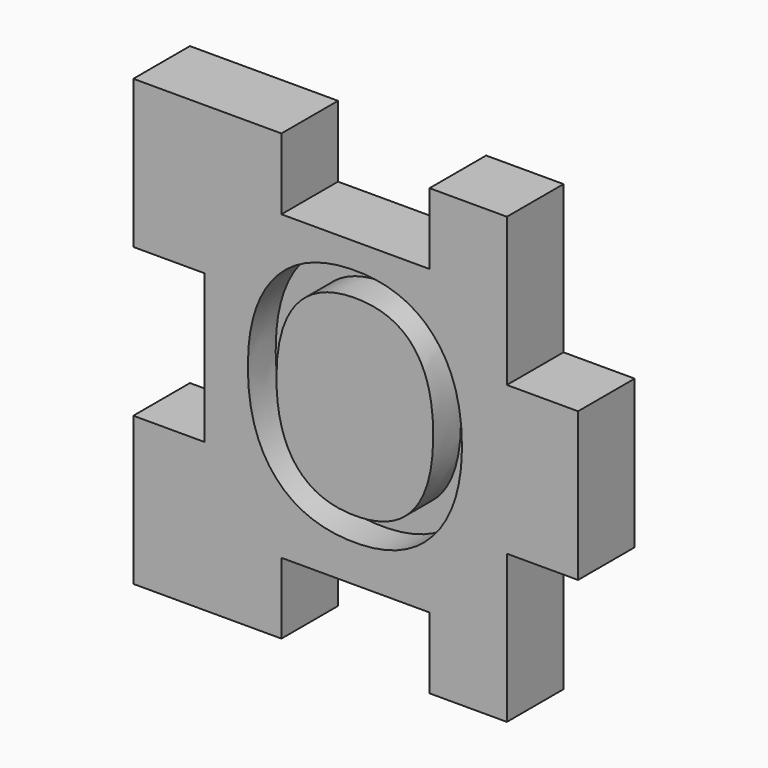
from build123d import *

# Parameters (mm, degrees)
F1_DEPTH     = 2.032
F2_TEXT_SIZE = 9.3656059094
F3_DEPTH     = 1


# Not quite as in the source:
# - a length typed as a fraction of an inch, garbled in the dataset ("3 / 203.2 mm" for 3/8 in), is restored
# - Text() gives the source's letters only with a copy of the font that has no kerning and outlines rounded to 1/6400 em; it was checked with that copy


with BuildPart() as f1:
    # F0 (on Front) → F1 (new body)
    with BuildSketch(Plane.XZ):
        Polygon((-10.9897290399, 29.0234165891), (-10.9897290399, 26.8898165891), (-10.9897290399, 24.7562165891), (-13.0344290399, 24.7562165891), (-13.0344290399, 20.5017165891), (-8.7799290399, 20.5017165891), (-8.7799290399, 22.5464165891), (-4.5254290399, 22.5464165891), (-4.5254290399, 20.5017165891), (-2.3029290399, 20.5017165891), (-2.3029290399, 24.7562165891), (-0.2582290399, 24.7562165891), (-0.2582290399, 29.0234165891), (-2.3029290399, 29.0234165891), (-2.3029290399, 33.2779165891), (-4.5254290399, 33.2779165891), (-4.5254290399, 31.2332165891), (-8.7799290399, 31.2332165891), (-8.7799290399, 33.2779165891), (-13.0344290399, 33.2779165891), (-13.0344290399, 29.0234165891), align=None)
    extrude(amount=F1_DEPTH)

    # F2 (on face) → F3 (cut)
    with BuildSketch(Plane.XZ.offset(2.032)):
        with Locations((-10.3177040399, 23.708849399)):
            Text('O', F2_TEXT_SIZE, font='Open Sans', text_align=(TextAlign.LEFT, TextAlign.BOTTOM))
    extrude(amount=-F3_DEPTH, mode=Mode.SUBTRACT)


solid = f1.part
